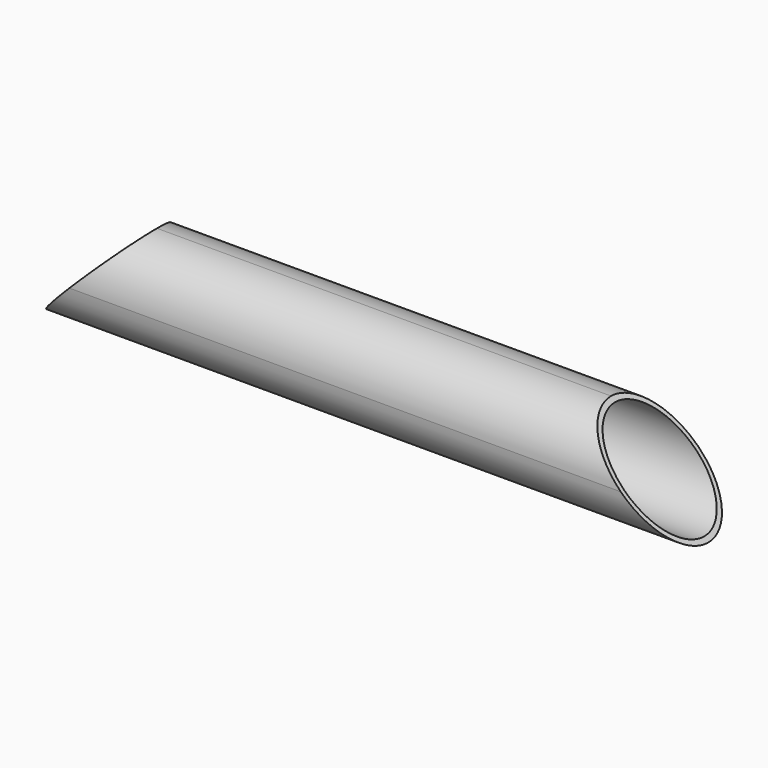
from build123d import *

# Parameters (mm, degrees)
F1_DEPTH = 6
F3_DEPTH = 6.001
F4_R     = 2.75
F5_DEPTH = 40.001
F6_R     = 2.99999
F7_DEPTH = 6.001


# Not quite as in the source:
# - a fillet or chamfer is up to 0.001 mm smaller than in the source, because OpenCascade refuses the exact size


with BuildPart() as f1:
    # F0 (on Top) → F1 (new body)
    with BuildSketch(Plane.XY):
        with BuildLine():
            Line((-8.5178157315, -13.6271222085), (-38.8432986429, -13.6271222085))
            Line((-38.8432986429, -13.6271222085), (-38.8432986429, -19.6271222085))
            Line((-38.8432986429, -19.6271222085), (-8.5178157315, -19.6271222085))
            ThreePointArc((-8.5178157315, -19.6271222085), (-11.5178157315, -16.6271222085), (-8.5178157315, -13.6271222085))
        make_face()
        with BuildLine():
            Line((1.1567013571, -13.6271222085), (-8.5178157315, -13.6271222085))
            ThreePointArc((-8.5178157315, -13.6271222085), (-6.3964953879, -14.5058018649), (-5.5178157315, -16.6271222085))
            ThreePointArc((-5.5178157315, -16.6271222085), (-6.3964953879, -18.748442552), (-8.5178157315, -19.6271222085))
            Line((-8.5178157315, -19.6271222085), (1.1567013571, -19.6271222085))
            Line((1.1567013571, -19.6271222085), (1.1567013571, -13.6271222085))
        make_face()
        with BuildLine():
            ThreePointArc((-5.5178157315, -16.6271222085), (-6.3964953879, -14.5058018649), (-8.5178157315, -13.6271222085))
            ThreePointArc((-8.5178157315, -13.6271222085), (-11.5178157315, -16.6271222085), (-8.5178157315, -19.6271222085))
            ThreePointArc((-8.5178157315, -19.6271222085), (-6.3964953879, -18.748442552), (-5.5178157315, -16.6271222085))
        make_face()
    extrude(amount=F1_DEPTH)

    # F2 (on face) → F3 (cut, through all)
    with BuildSketch(Plane.XZ.offset(19.6271222085)):
        Polygon((1.1567013571, 6), (-4.8432986429, 6), (1.1567013571, 0), align=None)
    extrude(amount=-F3_DEPTH, mode=Mode.SUBTRACT)

    # F4 (on face) → F5 (cut, through all)
    with BuildSketch(Plane(origin=(-38.8432986429, 0, 0), x_dir=(0, -1, 0), z_dir=(-1, 0, 0))):
        with Locations((16.6271222085, 3)):
            Circle(F4_R)
    extrude(amount=-F5_DEPTH, mode=Mode.SUBTRACT)

    # F6 (radius 3 in the source; OpenCascade refuses exactly that, so slightly less here)
    f6_edges = [f1.edges().sort_by_distance(p)[0] for p in [
        (-21.843299, -19.627122, 6),
        (-21.843299, -13.627122, 6),
        (-18.843299, -13.627122, 0),
        (-18.843299, -19.627122, 0),
    ]]
    fillet(f6_edges, radius=F6_R)

    # F2 (on face) → F7 (cut, through all)
    with BuildSketch(Plane.XZ.offset(19.6271222085)):
        Polygon((-38.8432986429, 0), (-32.8432986429, 6), (-38.8432986429, 6), align=None)
    extrude(amount=-F7_DEPTH, mode=Mode.SUBTRACT)


solid = f1.part
